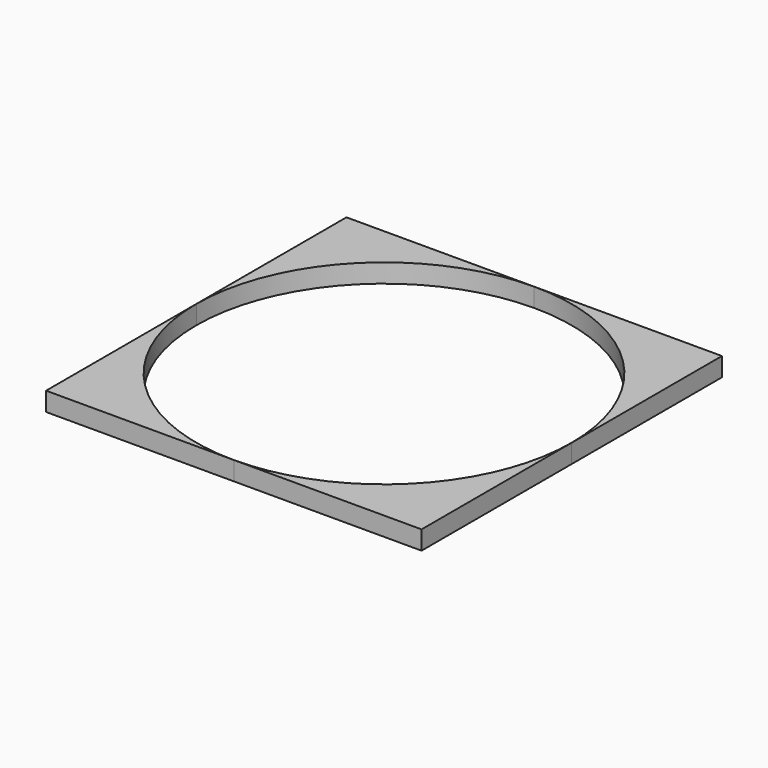
from build123d import *

# Parameters (mm, degrees)
F4_W     = 76.2
F4_H     = 76.2
F5_DEPTH = 3.81
F7_DEPTH = 101.346


# Not quite as in the source:
# - the program builds the solid bodies; features that only make, move or delete a surface that nothing else refers to are left out


with BuildPart() as f5:
    # F4 (on offset) → F5 (new body)
    with BuildSketch(Plane.XY.offset(-254)):
        Rectangle(F4_W, F4_H)
    extrude(amount=F5_DEPTH)

    # F6 (on face) → F7 (cut)
    with BuildSketch(Plane(origin=(0, 0, -254), x_dir=(1, 0, 0), z_dir=(0, 0, -1))):
        with BuildLine():
            ThreePointArc((0, -38.1), (26.9407683632, -26.9407683632), (38.1, 0))
            ThreePointArc((38.1, 0), (26.9407683632, 26.9407683632), (0, 38.1))
            ThreePointArc((0, 38.1), (-26.9407683632, 26.9407683632), (-38.1, 0))
            ThreePointArc((-38.1, 0), (-26.9407683632, -26.9407683632), (0, -38.1))
        make_face()
    extrude(amount=-F7_DEPTH, mode=Mode.SUBTRACT)


solid = f5.part
